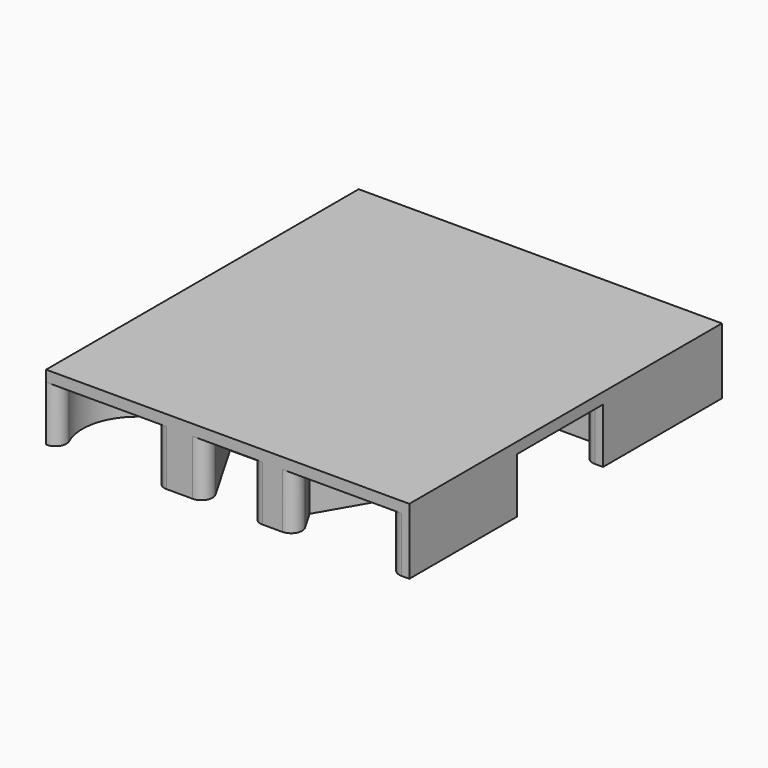
from build123d import *

# Parameters (mm, degrees)
F1_W     = 6.5
F1_H     = 19.5
F1_W_2   = 12.5
F1_H_2   = 5
F1_W_3   = 3.5
F2_DEPTH = 2
F3_DEPTH = 10
F4_R     = 2


# Not quite as in the source:
# - a feature names something its author has since deleted; it is built from what else it names


with BuildPart() as f2:
    # F1 (on Top) → F2 (new body)
    with BuildSketch(Plane.XY):
        with BuildLine():
            Line((-29.1414284285, 35.5), (-33, 35.5))
            Line((-33, 35.5), (-33, 8.5))
            Line((-33, 8.5), (-29.5, 8.5))
            Line((-29.5, 8.5), (-29.5, 13.5))
            Line((-29.5, 13.5), (-17, 13.5))
            Line((-17, 13.5), (-17, 8.5))
            Line((-17, 8.5), (-10.5, 8.5))
            Line((-10.5, 8.5), (-10.5, -11))
            Line((-10.5, -11), (-17, -11))
            Line((-17, -11), (-17, -16))
            Line((-17, -16), (-29.5, -16))
            Line((-29.5, -16), (-29.5, -11))
            Line((-29.5, -11), (-33, -11))
            Line((-33, -11), (-33, -35.5))
            Line((-33, -35.5), (-29.1414284285, -35.5))
            ThreePointArc((-29.1414284285, -35.5), (-25.7805896177, -19.2421848073), (-12, -28.5))
            ThreePointArc((-12, -28.5), (-12.7421848073, -32.2805896177), (-14.8585715715, -35.5))
            Line((-14.8585715715, -35.5), (-2.8867513459, -35.5))
            Line((-2.8867513459, -35.5), (-11.5, -20.581415713))
            Line((-11.5, -20.581415713), (11.5, -20.581415713))
            Line((11.5, -20.581415713), (2.8867513459, -35.5))
            Line((2.8867513459, -35.5), (13.3804538186, -35.5))
            Line((13.3804538186, -35.5), (9.4833395016, -28.75))
            Line((9.4833395016, -28.75), (15.1125046262, -19))
            Line((15.1125046262, -19), (26.3708348754, -19))
            Line((26.3708348754, -19), (32, -28.75))
            Line((32, -28.75), (28.102885683, -35.5))
            Line((28.102885683, -35.5), (33, -35.5))
            Line((33, -35.5), (33, -11))
            Line((33, -11), (29.5, -11))
            Line((29.5, -11), (29.5, -16))
            Line((29.5, -16), (17, -16))
            Line((17, -16), (17, -11))
            Line((17, -11), (10.5, -11))
            Line((10.5, -11), (10.5, 8.5))
            Line((10.5, 8.5), (17, 8.5))
            Line((17, 8.5), (17, 13.5))
            Line((17, 13.5), (29.5, 13.5))
            Line((29.5, 13.5), (29.5, 8.5))
            Line((29.5, 8.5), (33, 8.5))
            Line((33, 8.5), (33, 35.5))
            Line((33, 35.5), (28.2459666924, 35.5))
            ThreePointArc((28.2459666924, 35.5), (31.0197104752, 31.6460404129), (32, 27))
            ThreePointArc((32, 27), (15.8539595871, 16.4802895248), (12.7540333076, 35.5))
            Line((12.7540333076, 35.5), (3.3989794856, 35.5))
            ThreePointArc((3.3989794856, 35.5), (3.8476343915, 34.2856151892), (4, 33))
            Line((4, 33), (4, 20.5))
            Line((4, 20.5), (-7, 20.5))
            Line((-7, 20.5), (-7, 33))
            ThreePointArc((-7, 33), (-6.8476343915, 34.2856151892), (-6.3989794856, 35.5))
            Line((-6.3989794856, 35.5), (-14.8585715715, 35.5))
            ThreePointArc((-14.8585715715, 35.5), (-12.7421848073, 32.2805896177), (-12, 28.5))
            ThreePointArc((-12, 28.5), (-25.7805896177, 19.2421848073), (-29.1414284285, 35.5))
        make_face()
        with BuildLine():
            Line((-14.8585715715, 35.5), (-29.1414284285, 35.5))
            ThreePointArc((-29.1414284285, 35.5), (-25.7805896177, 19.2421848073), (-12, 28.5))
            ThreePointArc((-12, 28.5), (-12.7421848073, 32.2805896177), (-14.8585715715, 35.5))
        make_face()
        with BuildLine():
            ThreePointArc((-12, -28.5), (-25.7805896177, -19.2421848073), (-29.1414284285, -35.5))
            Line((-29.1414284285, -35.5), (-14.8585715715, -35.5))
            ThreePointArc((-14.8585715715, -35.5), (-12.7421848073, -32.2805896177), (-12, -28.5))
        make_face()
        Polygon((-11.5, -20.581415713), (-2.8867513459, -35.5), (2.8867513459, -35.5), (11.5, -20.581415713), align=None)
        with BuildLine():
            Line((28.2459666924, 35.5), (12.7540333076, 35.5))
            ThreePointArc((12.7540333076, 35.5), (15.8539595871, 16.4802895248), (32, 27))
            ThreePointArc((32, 27), (31.0197104752, 31.6460404129), (28.2459666924, 35.5))
        make_face()
        with BuildLine():
            Line((3.3989794856, 35.5), (-6.3989794856, 35.5))
            ThreePointArc((-6.3989794856, 35.5), (-6.8476343915, 34.2856151892), (-7, 33))
            Line((-7, 33), (4, 33))
            ThreePointArc((4, 33), (3.8476343915, 34.2856151892), (3.3989794856, 35.5))
        make_face()
        with BuildLine():
            Line((4, 33), (-7, 33))
            ThreePointArc((-7, 33), (-1.5, 27.5), (4, 33))
        make_face()
        with BuildLine():
            ThreePointArc((4, 33), (-1.5, 27.5), (-7, 33))
            Line((-7, 33), (-7, 20.5))
            Line((-7, 20.5), (4, 20.5))
            Line((4, 20.5), (4, 33))
        make_face()
        with Locations((13.75, -1.25)):
            Rectangle(F1_W, F1_H)
        with Locations((23.25, 11)):
            Rectangle(F1_W_2, F1_H_2)
        with Locations((23.25, -1.25)):
            Rectangle(F1_W_2, F1_H)
        with Locations((23.25, -13.5)):
            Rectangle(F1_W_2, F1_H_2)
        Polygon((9.4833395016, -28.75), (13.3804538186, -35.5), (28.102885683, -35.5), (32, -28.75), (26.3708348754, -19), (15.1125046262, -19), align=None)
        with Locations((31.25, -1.25)):
            Rectangle(F1_W_3, F1_H)
        with Locations((-31.25, -1.25)):
            Rectangle(F1_W_3, F1_H)
        with Locations((-23.25, -1.25)):
            Rectangle(F1_W_2, F1_H)
        with Locations((-13.75, -1.25)):
            Rectangle(F1_W, F1_H)
        with Locations((-23.25, 11)):
            Rectangle(F1_W_2, F1_H_2)
        with Locations((-23.25, -13.5)):
            Rectangle(F1_W_2, F1_H_2)
    extrude(amount=F2_DEPTH)

    # F1 (on Top) → F3 (join)
    with BuildSketch(Plane.XY):
        with BuildLine():
            Line((-29.1414284285, 35.5), (-33, 35.5))
            Line((-33, 35.5), (-33, 8.5))
            Line((-33, 8.5), (-29.5, 8.5))
            Line((-29.5, 8.5), (-29.5, 13.5))
            Line((-29.5, 13.5), (-17, 13.5))
            Line((-17, 13.5), (-17, 8.5))
            Line((-17, 8.5), (-10.5, 8.5))
            Line((-10.5, 8.5), (-10.5, -11))
            Line((-10.5, -11), (-17, -11))
            Line((-17, -11), (-17, -16))
            Line((-17, -16), (-29.5, -16))
            Line((-29.5, -16), (-29.5, -11))
            Line((-29.5, -11), (-33, -11))
            Line((-33, -11), (-33, -35.5))
            Line((-33, -35.5), (-29.1414284285, -35.5))
            ThreePointArc((-29.1414284285, -35.5), (-25.7805896177, -19.2421848073), (-12, -28.5))
            ThreePointArc((-12, -28.5), (-12.7421848073, -32.2805896177), (-14.8585715715, -35.5))
            Line((-14.8585715715, -35.5), (-2.8867513459, -35.5))
            Line((-2.8867513459, -35.5), (-11.5, -20.581415713))
            Line((-11.5, -20.581415713), (11.5, -20.581415713))
            Line((11.5, -20.581415713), (2.8867513459, -35.5))
            Line((2.8867513459, -35.5), (13.3804538186, -35.5))
            Line((13.3804538186, -35.5), (9.4833395016, -28.75))
            Line((9.4833395016, -28.75), (15.1125046262, -19))
            Line((15.1125046262, -19), (26.3708348754, -19))
            Line((26.3708348754, -19), (32, -28.75))
            Line((32, -28.75), (28.102885683, -35.5))
            Line((28.102885683, -35.5), (33, -35.5))
            Line((33, -35.5), (33, -11))
            Line((33, -11), (29.5, -11))
            Line((29.5, -11), (29.5, -16))
            Line((29.5, -16), (17, -16))
            Line((17, -16), (17, -11))
            Line((17, -11), (10.5, -11))
            Line((10.5, -11), (10.5, 8.5))
            Line((10.5, 8.5), (17, 8.5))
            Line((17, 8.5), (17, 13.5))
            Line((17, 13.5), (29.5, 13.5))
            Line((29.5, 13.5), (29.5, 8.5))
            Line((29.5, 8.5), (33, 8.5))
            Line((33, 8.5), (33, 35.5))
            Line((33, 35.5), (28.2459666924, 35.5))
            ThreePointArc((28.2459666924, 35.5), (31.0197104752, 31.6460404129), (32, 27))
            ThreePointArc((32, 27), (15.8539595871, 16.4802895248), (12.7540333076, 35.5))
            Line((12.7540333076, 35.5), (3.3989794856, 35.5))
            ThreePointArc((3.3989794856, 35.5), (3.8476343915, 34.2856151892), (4, 33))
            Line((4, 33), (4, 20.5))
            Line((4, 20.5), (-7, 20.5))
            Line((-7, 20.5), (-7, 33))
            ThreePointArc((-7, 33), (-6.8476343915, 34.2856151892), (-6.3989794856, 35.5))
            Line((-6.3989794856, 35.5), (-14.8585715715, 35.5))
            ThreePointArc((-14.8585715715, 35.5), (-12.7421848073, 32.2805896177), (-12, 28.5))
            ThreePointArc((-12, 28.5), (-25.7805896177, 19.2421848073), (-29.1414284285, 35.5))
        make_face()
    extrude(amount=-F3_DEPTH)

    # F4
    f4_edges = [f2.edges().sort_by_distance(p)[0] for p in [
        (-29.5, -11, -5),
        (-29.5, 8.5, -5),
        (-17, -11, -5),
        (-17, 8.5, -5),
        (17, -11, -5),
        (17, 8.5, -5),
        (29.5, -11, -5),
        (29.5, 8.5, -5),
        (-2.886751, -35.5, -5),
        (2.886751, -35.5, -5),
        (12.754033, 35.5, -5),
        (28.245967, 35.5, -5),
        (-29.141428, 35.5, -5),
        (-14.858572, 35.5, -5),
        (-29.141428, -35.5, -5),
        (-14.858572, -35.5, -5),
        (13.380454, -35.5, -5),
        (28.102886, -35.5, -5),
    ]]
    fillet(f4_edges, radius=F4_R)


solid = f2.part
